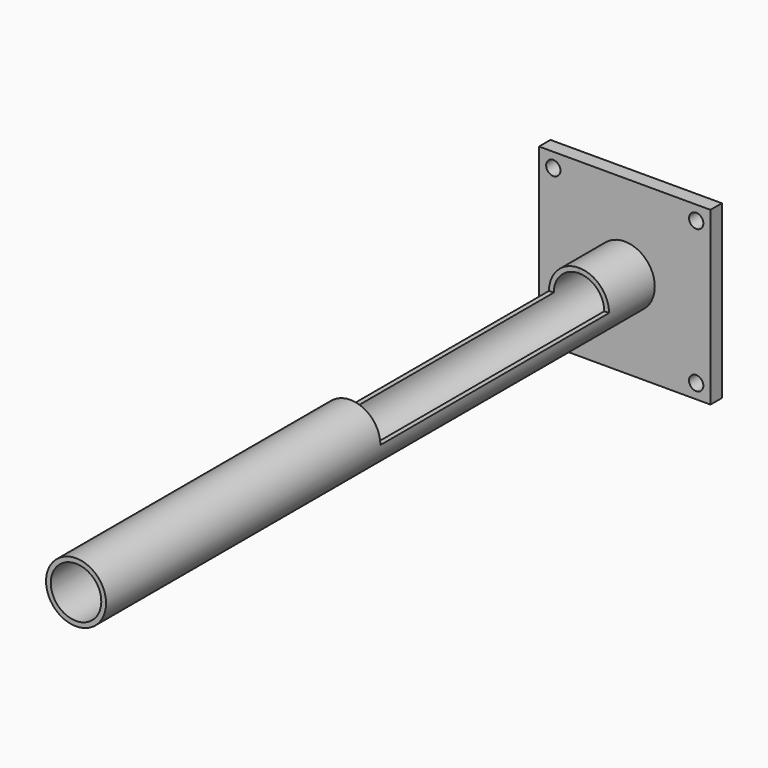
from build123d import *

# Parameters (mm, degrees)
F0_R          = 13.335
F0_R_2        = 11.2268
F1_DEPTH      = 304.8
F2_W          = 76.2
F2_H          = 76.2
F2_R          = 11.2268
F3_DEPTH      = 6.35
F4_W          = 127
F4_H          = 30.226
F5_DEPTH      = 38.101
F5_DEPTH_BACK = 38.101
F6_R          = 3.175
F7_DEPTH      = 6.351


# Not quite as in the source:
# - a length typed as a fraction of an inch, garbled in the dataset ("3 / 203.2 mm" for 3/8 in), is restored


with BuildPart() as f1:
    # F0 (on Front) → F1 (new body)
    with BuildSketch(Plane.XZ):
        Circle(F0_R)
        Circle(F0_R_2, mode=Mode.SUBTRACT)
    extrude(amount=F1_DEPTH)

    # F2 (on face) → F3 (join)
    with BuildSketch(Plane(origin=(0, 0, 0), x_dir=(-1, 0, 0), z_dir=(0, 1, 0))):
        Rectangle(F2_W, F2_H)
        Circle(F2_R, mode=Mode.SUBTRACT)
    extrude(amount=F3_DEPTH)

    # F4 (on Right) → F5 (cut, two sides)
    with BuildSketch(Plane.YZ) as f5_sk:
        with Locations((-88.9, 15.113)):
            Rectangle(F4_W, F4_H)
    extrude(amount=-F5_DEPTH, mode=Mode.SUBTRACT)
    extrude(f5_sk.sketch, amount=F5_DEPTH_BACK, mode=Mode.SUBTRACT)

    # F6 (on face) → F7 (cut, through all)
    with BuildSketch(Plane.XZ):
        with Locations((-31.75, 31.75)):
            Circle(F6_R)
        with Locations((-31.75, -31.75)):
            Circle(F6_R)
        with Locations((31.75, 31.75)):
            Circle(F6_R)
        with Locations((31.75, -31.75)):
            Circle(F6_R)
    extrude(amount=-F7_DEPTH, mode=Mode.SUBTRACT)


solid = f1.part
